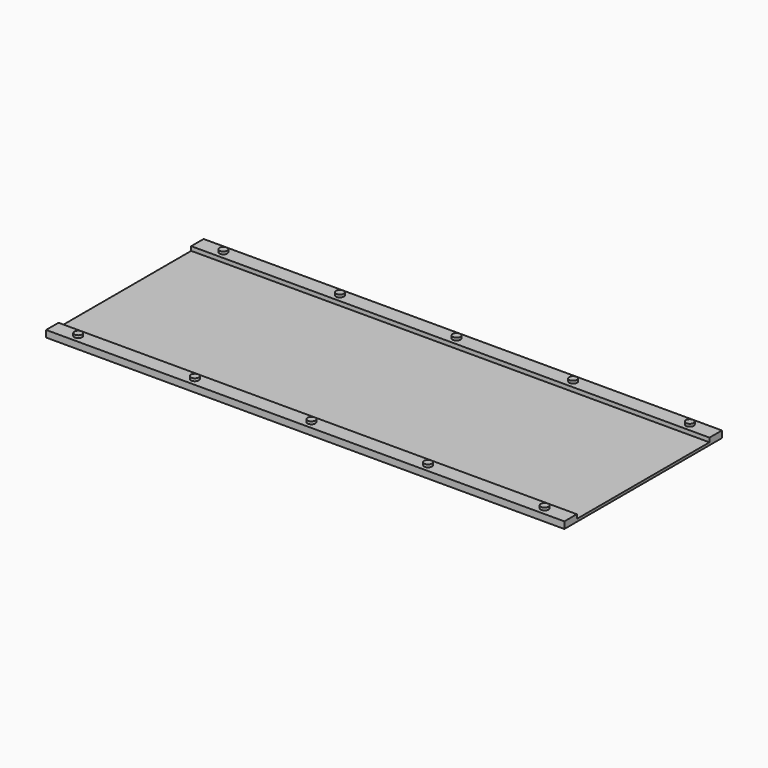
from build123d import *

# Parameters (mm, degrees)
F0_W     = 100
F0_H     = 38
F1_DEPTH = 0.5
F2_W     = 100
F2_H     = 3
F3_DEPTH = 0.8
F4_R     = 0.75
F5_DEPTH = 0.5
F6_R     = 0.75
F7_DEPTH = 0.5


# Not quite as in the source:
# - a feature names something its author has since deleted; it is built from what else it names


with BuildPart() as f1:
    # F0 (on Top) → F1 (new body)
    with BuildSketch(Plane.XY):
        with Locations((-50, 0)):
            Rectangle(F0_W, F0_H)
    extrude(amount=-F1_DEPTH)

    # F2 (on face) → F3 (join)
    with BuildSketch(Plane.XY):
        with Locations((-50, 17.5)):
            Rectangle(F2_W, F2_H)
        with Locations((-50, -17.5)):
            Rectangle(F2_W, F2_H)
    extrude(amount=F3_DEPTH)

    # F4 (on face) → F5 (join)
    with BuildSketch(Plane.XY.offset(0.8)):
        with Locations((-95, 17.5)):
            Circle(F4_R)
        with Locations((-72.5, 17.5)):
            Circle(F4_R)
        with Locations((-50, 17.5)):
            Circle(F4_R)
        with Locations((-27.5, 17.5)):
            Circle(F4_R)
        with Locations((-5, 17.5)):
            Circle(F4_R)
    extrude(amount=F5_DEPTH)

    # F6 (on face) → F7 (join)
    with BuildSketch(Plane.XY.offset(0.8)):
        with Locations((-95, -17.5)):
            Circle(F6_R)
        with Locations((-72.5, -17.5)):
            Circle(F6_R)
        with Locations((-50, -17.5)):
            Circle(F6_R)
        with Locations((-27.5, -17.5)):
            Circle(F6_R)
        with Locations((-5, -17.5)):
            Circle(F6_R)
    extrude(amount=F7_DEPTH)


solid = f1.part
